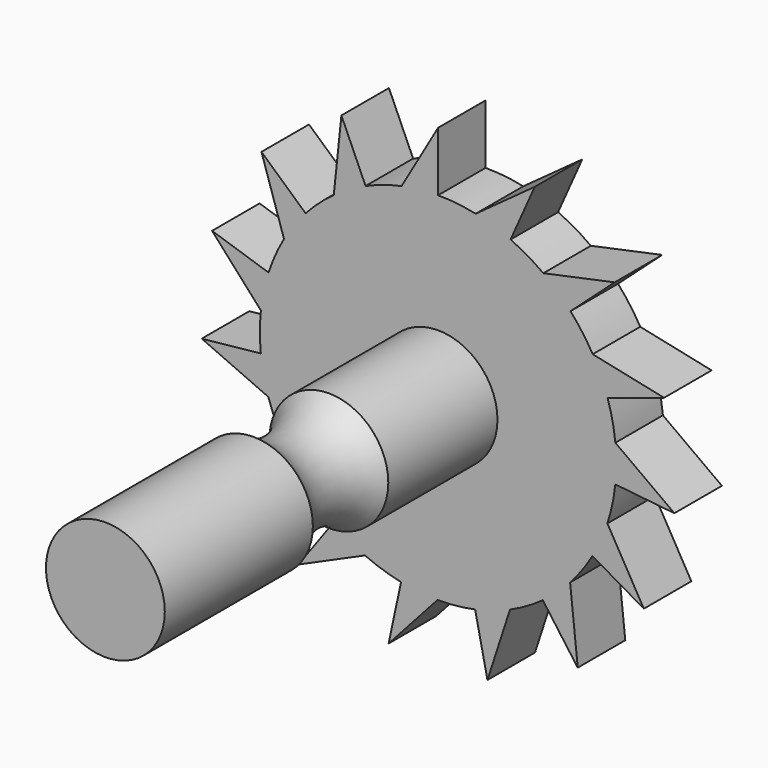
from build123d import *

# Parameters (mm, degrees)
F0_R            = 38.1
F1_DEPTH        = 12.7
F3_DEPTH        = 12.7
F3_COPIES_COUNT = 15
F4_R            = 12.7
F5_DEPTH        = 101.6


# Not quite as in the source:
# - a pattern or mirror of a feature is missing from the dataset's text; its kind, count and spacing are read off the source's solid


with BuildPart() as f1:
    # F0 (on Front) → F1 (new body)
    with BuildSketch(Plane.XZ):
        Circle(F0_R)
    extrude(amount=F1_DEPTH)

    # F2 (on Front) → F3 (join, through all)
    with BuildSketch(Plane.XZ):
        Polygon((0, 50.8), (-7.798013599, 37.2934442484), (0, 38.1), align=None)
    f3 = extrude(amount=F3_DEPTH)

    # F3_copies: F3 ×15 about axis
    f3_copies_axis = Axis((0, 0, 0), (0, 1, 0))
    for i in range(1, F3_COPIES_COUNT):
        add(f3.rotate(f3_copies_axis, i * 360 / F3_COPIES_COUNT))

    # F4 (on Front) → F5 (join)
    with BuildSketch(Plane.XZ):
        Circle(F4_R)
    extrude(amount=F5_DEPTH)

    # F6 (on Right) → F7 (revolve, cut)
    with BuildSketch(Plane.YZ):
        with BuildLine():
            Line((-38.1, 17.78), (-65.8081287712, 17.78))
            ThreePointArc((-65.8081287712, 17.78), (-51.9540643856, 8.89), (-38.1, 17.78))
        make_face()
    revolve(axis=Axis((0, 0, 0), (0, 1, 0)), mode=Mode.SUBTRACT)


solid = f1.part
